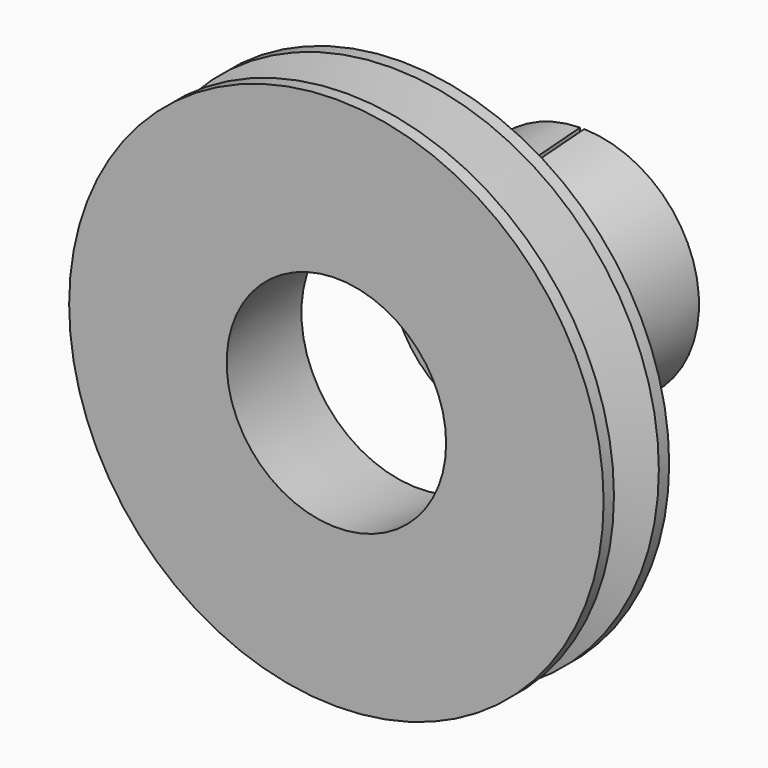
from build123d import *

# Parameters (mm, degrees)
F2_R      = 26.79
F3_DEPTH  = 25
F3_TAPER  = -4
F5_R      = 26.79
F6_DEPTH  = 25
F6_TAPER  = -4
F7_R      = 17.5
F8_DEPTH  = 25
F10_DEPTH = 25


with BuildPart() as f1:
    # F0 (on Right) → F1 (revolve)
    with BuildSketch(Plane.YZ):
        Polygon((0, 65.25), (0, 0), (25, 0), (25, 46), (20, 46), (20, 65.25), (16.85, 65.25), (13.4258163677, 54.05), (6.5741836323, 54.05), (3.15, 65.25), align=None)
    revolve(axis=Axis((0, 12.5, 0), (0, -1, 0)))

    # F2 (on face) → F3 (cut)
    with BuildSketch(Plane.XZ):
        Circle(F2_R)
    extrude(amount=-F3_DEPTH, taper=F3_TAPER, mode=Mode.SUBTRACT)


with BuildPart() as f6:
    # F5 (on offset) → F6 (new body)
    with BuildSketch(Plane(origin=(0, 50, 0), x_dir=(-1, 0, 0), z_dir=(0, 1, 0))):
        Circle(F5_R)
    extrude(amount=F6_DEPTH, taper=F6_TAPER)

    # F7 (on face) → F8 (cut, through all)
    with BuildSketch(Plane(origin=(0, 75, 0), x_dir=(-1, 0, 0), z_dir=(0, 1, 0))):
        Circle(F7_R)
    extrude(amount=-F8_DEPTH, mode=Mode.SUBTRACT)

    # F9 (on face) → F10 (cut, through all)
    with BuildSketch(Plane(origin=(0, 75, 0), x_dir=(-1, 0, 0), z_dir=(0, 1, 0))):
        with BuildLine():
            Line((0.5, -21.1339745962), (0.5, 30))
            Line((0.5, 30), (-0.5, 30))
            Line((-0.5, 30), (-0.5, -21.1339745962))
            ThreePointArc((-0.5, -21.1339745962), (0, -21), (0.5, -21.1339745962))
        make_face()
        with BuildLine():
            ThreePointArc((1, -22), (0.8660254038, -21.5), (0.5, -21.1339745962))
            Line((0.5, -21.1339745962), (0.5, -22))
            Line((0.5, -22), (-0.5, -22))
            Line((-0.5, -22), (-0.5, -21.1339745962))
            ThreePointArc((-0.5, -21.1339745962), (-0.5, -22.8660254038), (1, -22))
        make_face()
        with BuildLine():
            Line((0.5, -22), (0.5, -21.1339745962))
            ThreePointArc((0.5, -21.1339745962), (0, -21), (-0.5, -21.1339745962))
            Line((-0.5, -21.1339745962), (-0.5, -22))
            Line((-0.5, -22), (0.5, -22))
        make_face()
    extrude(amount=-F10_DEPTH, mode=Mode.SUBTRACT)


solid = Compound([f1.part, f6.part])
